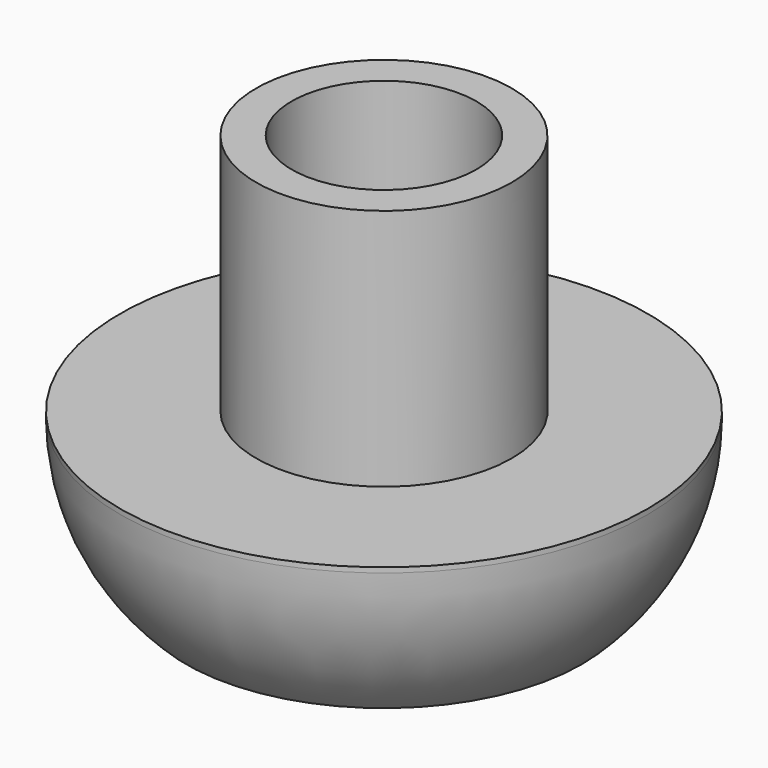
from build123d import *

# Parameters (mm, degrees)
F0_R     = 6.35
F1_DEPTH = 3.81
F2_R     = 3.0734
F3_DEPTH = 5.842
F4_R     = 2.2225
F5_DEPTH = 9.653
F6_SIZE2 = 2.54
F6_SIZE  = 2.54


# Not quite as in the source:
# - a fillet or chamfer that OpenCascade refuses, or shapes differently, is made with other operations: its cross-section is extruded or revolved along the edge and cut away or added


with BuildPart() as f1:
    # F0 (on Top) → F1 (new body)
    with BuildSketch(Plane.XY):
        Circle(F0_R)
    extrude(amount=F1_DEPTH)

    # F2 (on face) → F3 (join)
    with BuildSketch(Plane.XY.offset(3.81)):
        Circle(F2_R)
    extrude(amount=F3_DEPTH)

    # F4 (on face) → F5 (cut, through all)
    with BuildSketch(Plane.XY.offset(9.652)):
        Circle(F4_R)
    extrude(amount=-F5_DEPTH, mode=Mode.SUBTRACT)

    # F6
    f6_edges = [f1.edges().sort_by_distance(p)[0] for p in [
        (-2.2225, 0, 0),
    ]]
    chamfer(f6_edges, length=F6_SIZE, length2=F6_SIZE2)

    # F7: fillet of radius 5.08 on 1 edges, made by hand

    # F7_s1 → F7_t2 (revolve, cut)
    with BuildSketch(Plane.XZ):
        with BuildLine():
            ThreePointArc((4.7625, 0), (5.93627796, 1.6809703231), (6.35, 3.6890166373))
            Line((6.35, 3.6890166373), (6.35, 0))
            Line((6.35, 0), (4.7625, 0))
        make_face()
    revolve(axis=Axis((0, 0, 0), (0, 0, 1)), mode=Mode.SUBTRACT)


solid = f1.part
